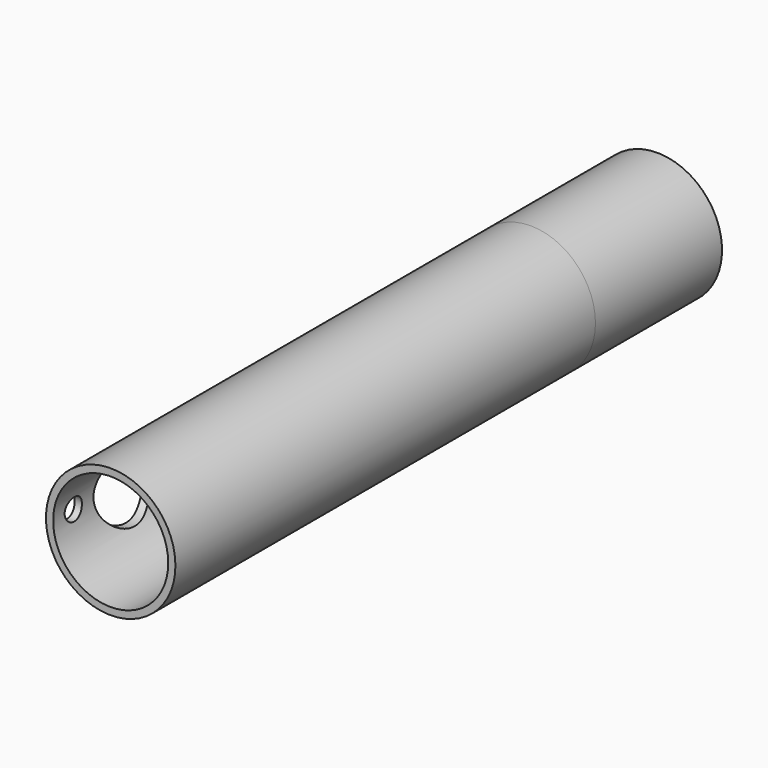
from build123d import *

# Parameters (mm, degrees)
F3_R      = 4.5
F4_DEPTH  = 27.5
F8_DEPTH  = 27.5
F6_R      = 4.5
F6_R_2    = 4
F9_DEPTH  = 9
F7_R      = 4.5
F7_R_2    = 4
F10_DEPTH = 11
F11_R     = 2.5
F11_R_2   = 0.75
F12_DEPTH = 4.501


# Not quite as in the source:
# - ends of sketch curves that miss each other by under 0.0002 mm in the source are joined


with BuildPart() as f4:
    # F3 (on Front) → F4 (new body)
    with BuildSketch(Plane.XZ):
        Circle(F3_R)
    extrude(amount=F4_DEPTH)

    # F5 (on face) → F8 (cut, through all)
    with BuildSketch(Plane.XZ.offset(27.5)):
        with BuildLine():
            Line((-1.25, -3.8), (0, -3.8))
            Line((0, -3.8), (1.25, -3.8))
            Line((1.25, -3.8), (1.25, -3.7))
            ThreePointArc((1.25, -3.7), (1.3085786438, -3.5585786438), (1.45, -3.5))
            Line((1.45, -3.5), (2, -3.5))
            Line((2, -3.5), (2, -3.05))
            ThreePointArc((2, -3.05), (2.0585786438, -2.9085786438), (2.2, -2.85))
            Line((2.2, -2.85), (3.15, -2.85))
            Line((3.15, -2.85), (3.15, -2.15))
            Line((3.15, -2.15), (2.2, -2.15))
            ThreePointArc((2.2, -2.15), (2.0585786438, -2.0914213562), (2, -1.95))
            Line((2, -1.95), (2, -1.887459))
            ThreePointArc((2, -1.887459), (2.1033535752, -1.771554046), (2.2, -1.65))
            Line((2.2, -1.65), (3.75, -1.65))
            Line((3.75, -1.65), (3.75, 0))
            Line((3.75, 0), (3.75, 1.65))
            Line((3.75, 1.65), (2.2, 1.65))
            ThreePointArc((2.2, 1.65), (2.1033535752, 1.771554046), (1.9999998047, 1.8874588157))
            Line((1.9999998047, 1.8874588157), (2, 1.95))
            ThreePointArc((2, 1.95), (2.0585786438, 2.0914213562), (2.2, 2.15))
            Line((2.2, 2.15), (3.15, 2.15))
            Line((3.15, 2.15), (3.15, 2.85))
            Line((3.15, 2.85), (2.2, 2.85))
            ThreePointArc((2.2, 2.85), (2.0585786438, 2.9085786438), (2, 3.05))
            Line((2, 3.05), (2, 3.5))
            Line((2, 3.5), (1.45, 3.5))
            ThreePointArc((1.45, 3.5), (1.3085786438, 3.5585786438), (1.25, 3.7))
            Line((1.25, 3.7), (1.25, 3.8))
            Line((1.25, 3.8), (0, 3.8))
            Line((0, 3.8), (-1.25, 3.8))
            Line((-1.25, 3.8), (-1.25, 3.7))
            ThreePointArc((-1.25, 3.7), (-1.3085786438, 3.5585786438), (-1.45, 3.5))
            Line((-1.45, 3.5), (-2, 3.5))
            Line((-2, 3.5), (-2, 3.05))
            ThreePointArc((-2, 3.05), (-2.0585786438, 2.9085786438), (-2.2, 2.85))
            Line((-2.2, 2.85), (-3.15, 2.85))
            Line((-3.15, 2.85), (-3.15, 2.15))
            Line((-3.15, 2.15), (-2.2, 2.15))
            ThreePointArc((-2.2, 2.15), (-2.0585786438, 2.0914213562), (-2, 1.95))
            Line((-2, 1.95), (-2, 1.887459))
            ThreePointArc((-2, 1.887459), (-2.1033535752, 1.771554046), (-2.2, 1.65))
            Line((-2.2, 1.65), (-3.75, 1.65))
            Line((-3.75, 1.65), (-3.75, 0))
            Line((-3.75, 0), (-3.75, -1.65))
            Line((-3.75, -1.65), (-2.2, -1.65))
            ThreePointArc((-2.2, -1.65), (-2.1033535752, -1.771554046), (-1.9999998047, -1.8874588157))
            Line((-1.9999998047, -1.8874588157), (-2, -1.95))
            ThreePointArc((-2, -1.95), (-2.0585786438, -2.0914213562), (-2.2, -2.15))
            Line((-2.2, -2.15), (-3.15, -2.15))
            Line((-3.15, -2.15), (-3.15, -2.85))
            Line((-3.15, -2.85), (-2.2, -2.85))
            ThreePointArc((-2.2, -2.85), (-2.0585786438, -2.9085786438), (-2, -3.05))
            Line((-2, -3.05), (-2, -3.5))
            Line((-2, -3.5), (-1.45, -3.5))
            ThreePointArc((-1.45, -3.5), (-1.3085786438, -3.5585786438), (-1.25, -3.7))
            Line((-1.25, -3.7), (-1.25, -3.8))
        make_face()
    extrude(amount=-F8_DEPTH, mode=Mode.SUBTRACT)

    # F6 (on face) → F9 (join)
    with BuildSketch(Plane.XZ.offset(27.5)):
        Circle(F6_R)
        Circle(F6_R_2, mode=Mode.SUBTRACT)
    extrude(amount=F9_DEPTH)

    # F7 (on face) → F10 (join)
    with BuildSketch(Plane(origin=(0, 0, 0), x_dir=(-1, 0, 0), z_dir=(0, 1, 0))):
        Circle(F7_R)
        Circle(F7_R_2, mode=Mode.SUBTRACT)
    extrude(amount=F10_DEPTH)

    # F11 (on Right) → F12 (cut, through all)
    with BuildSketch(Plane.YZ):
        with Locations((-30.5, 0)):
            Circle(F11_R)
        with Locations((-34.75, 0)):
            Circle(F11_R_2)
    extrude(amount=-F12_DEPTH, mode=Mode.SUBTRACT)


solid = f4.part
